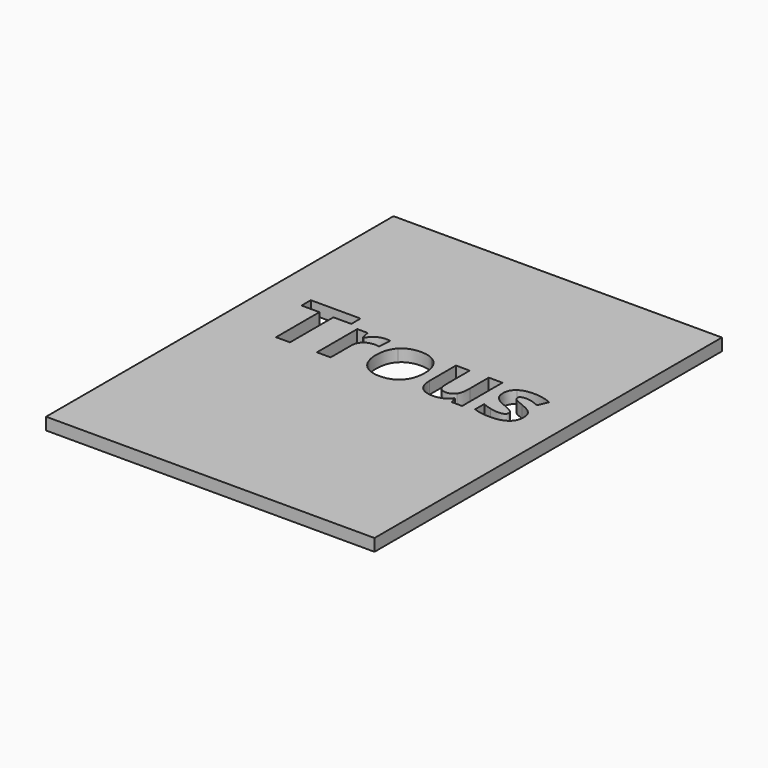
from build123d import *

# Parameters (mm, degrees)
F1_DEPTH = 10


# Not quite as in the source:
# - a feature names something its author has since deleted; it is built from what else it names


with BuildPart() as f1:
    # F0 (on Top) → F1 (new body)
    with BuildSketch(Plane.XY):
        Polygon((-135, 145.3171813515), (-135, -111.8657903795), (-105, -111.8657903795), (-105, 115.3171813515), (0, 115.3171813515), (0, 145.3171813515), align=None)
        Polygon((81.1492523154, -181.6828186485), (81.1492523154, -211.6828186485), (135, -211.6828186485), (135, -33.1828186485), (105, -33.1828186485), (105, -181.6828186485), align=None)
        Polygon((105, -33.1828186485), (135, -33.1828186485), (135, 145.3171813515), (0, 145.3171813515), (0, 115.3171813515), (105, 115.3171813515), (105, -20.8807700001), align=None)
        Polygon((-135, -111.8657903795), (-135, -211.6828186485), (81.1492523154, -211.6828186485), (81.1492523154, -181.6828186485), (-105, -181.6828186485), (-105, -111.8657903795), align=None)
        Polygon((-105, -181.6828186485), (81.1492523154, -181.6828186485), (105, -181.6828186485), (105, -33.1828186485), (105, -20.8807700001), (105, 115.3171813515), (0, 115.3171813515), (-105, 115.3171813515), (-105, -111.8657903795), align=None)
        Polygon((-77.2907613296, 11.4150706229), (-77.2907613296, -33.1828186485), (-88.7750437384, -33.1828186485), (-88.7750437384, 11.4150706229), (-103.4829843671, 11.4150706229), (-103.4829843671, 20.9675284366), (-62.5946723856, 20.9675284366), (-62.5946723856, 11.4150706229), align=None, mode=Mode.SUBTRACT)
        with BuildLine():
            add(Edge.make_bspline(
                [(-39.1698177098, 6.8699495664), (-35.892826909, 8.9973269579), (-32.0410294035, 8.9973269579)],
                knots=[0, 0, 0, 1, 1, 1], degree=2))
            add(Edge.make_bspline(
                [(-32.0410294035, 8.9973269579), (-29.7418025848, 8.9973269579), (-28.2247869519, 8.6654797882)],
                knots=[0, 0, 0, 1, 1, 1], degree=2))
            Line((-28.2247869519, 8.6654797882), (-29.0781082454, -1.9180745884))
            add(Edge.make_bspline(
                [(-29.0781082454, -1.9180745884), (-30.4529036627, -1.5506723648), (-32.4084316271, -1.5506723648)],
                knots=[0, 0, 0, 1, 1, 1], degree=2))
            add(Edge.make_bspline(
                [(-32.4084316271, -1.5506723648), (-37.8127998194, -1.5506723648), (-40.8349794006, -4.3298924111)],
                knots=[0, 0, 0, 1, 1, 1], degree=2))
            add(Edge.make_bspline(
                [(-40.8349794006, -4.3298924111), (-43.8571589819, -7.1091124574), (-43.8571589819, -12.1105233722)],
                knots=[0, 0, 0, 1, 1, 1], degree=2))
            Line((-43.8571589819, -12.1105233722), (-43.8571589819, -33.1828186485))
            Line((-43.8571589819, -33.1828186485), (-55.1518144365, -33.1828186485))
            Line((-55.1518144365, -33.1828186485), (-55.1518144365, 8.2269674568))
            Line((-55.1518144365, 8.2269674568), (-46.5948981319, 8.2269674568))
            Line((-46.5948981319, 8.2269674568), (-44.9238105988, 1.258176893))
            Line((-44.9238105988, 1.258176893), (-44.3786331057, 1.258176893))
            add(Edge.make_bspline(
                [(-44.3786331057, 1.258176893), (-42.4468085106, 4.7425721749), (-39.1698177098, 6.8699495664)],
                knots=[0, 0, 0, 1, 1, 1], degree=2))
        make_face(mode=Mode.SUBTRACT)
        with BuildLine():
            add(Edge.make_bspline(
                [(14.4768327784, -1.0351240833), (16.9182798126, -5.8883889403), (16.9182798126, -12.406815488)],
                knots=[0, 0, 0, 1, 1, 1], degree=2))
            add(Edge.make_bspline(
                [(16.9182798126, -12.406815488), (16.9182798126, -22.5163024794), (11.5850217281, -28.2228886299)],
                knots=[0, 0, 0, 1, 1, 1], degree=2))
            add(Edge.make_bspline(
                [(11.5850217281, -28.2228886299), (6.2517636435, -33.9294747803), (-3.2651391162, -33.9294747803)],
                knots=[0, 0, 0, 1, 1, 1], degree=2))
            add(Edge.make_bspline(
                [(-3.2651391162, -33.9294747803), (-9.2265364863, -33.9294747803), (-13.7835092274, -31.3161783189)],
                knots=[0, 0, 0, 1, 1, 1], degree=2))
            add(Edge.make_bspline(
                [(-13.7835092274, -31.3161783189), (-18.3404819685, -28.7028818575), (-20.7819290028, -23.8140619466)],
                knots=[0, 0, 0, 1, 1, 1], degree=2))
            add(Edge.make_bspline(
                [(-20.7819290028, -23.8140619466), (-23.223376037, -18.9252420358), (-23.223376037, -12.406815488)],
                knots=[0, 0, 0, 1, 1, 1], degree=2))
            add(Edge.make_bspline(
                [(-23.223376037, -12.406815488), (-23.223376037, -2.2617734428), (-17.9315988487, 3.3677767576)],
                knots=[0, 0, 0, 1, 1, 1], degree=2))
            add(Edge.make_bspline(
                [(-17.9315988487, 3.3677767576), (-12.6398216604, 8.9973269579), (-3.0399571082, 8.9973269579)],
                knots=[0, 0, 0, 1, 1, 1], degree=2))
            add(Edge.make_bspline(
                [(-3.0399571082, 8.9973269579), (2.9214402619, 8.9973269579), (7.478413003, 6.4077338658)],
                knots=[0, 0, 0, 1, 1, 1], degree=2))
            add(Edge.make_bspline(
                [(7.478413003, 6.4077338658), (12.0353857441, 3.8181407736), (14.4768327784, -1.0351240833)],
                knots=[0, 0, 0, 1, 1, 1], degree=2))
        make_face(mode=Mode.SUBTRACT)
        with BuildLine():
            Line((64.2539082341, -33.1828186485), (55.5903267679, -33.1828186485))
            Line((55.5903267679, -33.1828186485), (54.0733111349, -27.8851156178))
            Line((54.0733111349, -27.8851156178), (53.4807269033, -27.8851156178))
            add(Edge.make_bspline(
                [(53.4807269033, -27.8851156178), (51.6674191546, -30.7769266681), (48.3311699306, -32.3532007242)],
                knots=[0, 0, 0, 1, 1, 1], degree=2))
            add(Edge.make_bspline(
                [(48.3311699306, -32.3532007242), (44.9949207066, -33.9294747803), (40.7401659236, -33.9294747803)],
                knots=[0, 0, 0, 1, 1, 1], degree=2))
            add(Edge.make_bspline(
                [(40.7401659236, -33.9294747803), (33.4395281901, -33.9294747803), (29.7358767425, -30.0184188517)],
                knots=[0, 0, 0, 1, 1, 1], degree=2))
            add(Edge.make_bspline(
                [(29.7358767425, -30.0184188517), (26.0322252949, -26.107362923), (26.0322252949, -18.7711701356)],
                knots=[0, 0, 0, 1, 1, 1], degree=2))
            Line((26.0322252949, -18.7711701356), (26.0322252949, 8.2269674568))
            Line((26.0322252949, 8.2269674568), (37.3268807495, 8.2269674568))
            Line((37.3268807495, 8.2269674568), (37.3268807495, -15.9623208777))
            add(Edge.make_bspline(
                [(37.3268807495, -15.9623208777), (37.3268807495, -20.4422576688), (38.9209323325, -22.6822260643)],
                knots=[0, 0, 0, 1, 1, 1], degree=2))
            add(Edge.make_bspline(
                [(38.9209323325, -22.6822260643), (40.5149839156, -24.9221944598), (43.9993791975, -24.9221944598)],
                knots=[0, 0, 0, 1, 1, 1], degree=2))
            add(Edge.make_bspline(
                [(43.9993791975, -24.9221944598), (48.7400530504, -24.9221944598), (50.8496529149, -21.7577946629)],
                knots=[0, 0, 0, 1, 1, 1], degree=2))
            add(Edge.make_bspline(
                [(50.8496529149, -21.7577946629), (52.9592527795, -18.5933948661), (52.9592527795, -11.2572020787)],
                knots=[0, 0, 0, 1, 1, 1], degree=2))
            Line((52.9592527795, -11.2572020787), (52.9592527795, 8.2269674568))
            Line((52.9592527795, 8.2269674568), (64.2539082341, 8.2269674568))
            Line((64.2539082341, 8.2269674568), (64.2539082341, -33.1828186485))
        make_face(mode=Mode.SUBTRACT)
        with BuildLine():
            add(Edge.make_bspline(
                [(103.9214966985, -15.5889928118), (105, -17.8111836804), (105, -20.8807700001)],
                knots=[0, 0, 0, 1, 1, 1], degree=2))
            add(Edge.make_bspline(
                [(105, -20.8807700001), (105, -27.2569763323), (100.5733957898, -30.5932255563)],
                knots=[0, 0, 0, 1, 1, 1], degree=2))
            add(Edge.make_bspline(
                [(100.5733957898, -30.5932255563), (96.1467915797, -33.9294747803), (87.3291382132, -33.9294747803)],
                knots=[0, 0, 0, 1, 1, 1], degree=2))
            add(Edge.make_bspline(
                [(87.3291382132, -33.9294747803), (82.8136463683, -33.9294747803), (79.6255432022, -33.3131871794)],
                knots=[0, 0, 0, 1, 1, 1], degree=2))
            add(Edge.make_bspline(
                [(79.6255432022, -33.3131871794), (76.4374400361, -32.6968995786), (73.6641458322, -31.5117311153)],
                knots=[0, 0, 0, 1, 1, 1], degree=2))
            Line((73.6641458322, -31.5117311153), (73.6641458322, -22.1844553097))
            add(Edge.make_bspline(
                [(73.6641458322, -22.1844553097), (76.8048422597, -23.6659158887), (80.7514532423, -24.6673832402)],
                knots=[0, 0, 0, 1, 1, 1], degree=2))
            add(Edge.make_bspline(
                [(80.7514532423, -24.6673832402), (84.6980642248, -25.6688505916), (87.6965404368, -25.6688505916)],
                knots=[0, 0, 0, 1, 1, 1], degree=2))
            add(Edge.make_bspline(
                [(87.6965404368, -25.6688505916), (93.847564761, -25.6688505916), (93.847564761, -22.1133452019)],
                knots=[0, 0, 0, 1, 1, 1], degree=2))
            add(Edge.make_bspline(
                [(93.847564761, -22.1133452019), (93.847564761, -20.7741048385), (93.0297985214, -19.9385610719)],
                knots=[0, 0, 0, 1, 1, 1], degree=2))
            add(Edge.make_bspline(
                [(93.0297985214, -19.9385610719), (92.2120322817, -19.1030173053), (90.2150234212, -18.048217373)],
                knots=[0, 0, 0, 1, 1, 1], degree=2))
            add(Edge.make_bspline(
                [(90.2150234212, -18.048217373), (88.2180145606, -16.9934174408), (84.887691179, -15.5949186541)],
                knots=[0, 0, 0, 1, 1, 1], degree=2))
            add(Edge.make_bspline(
                [(84.887691179, -15.5949186541), (80.1114622721, -13.5919839513), (77.8655680343, -11.8853413642)],
                knots=[0, 0, 0, 1, 1, 1], degree=2))
            add(Edge.make_bspline(
                [(77.8655680343, -11.8853413642), (75.6196737965, -10.1786987772), (74.6063547604, -7.9742854356)],
                knots=[0, 0, 0, 1, 1, 1], degree=2))
            add(Edge.make_bspline(
                [(74.6063547604, -7.9742854356), (73.5930357244, -5.7698720939), (73.5930357244, -2.5580655586)],
                knots=[0, 0, 0, 1, 1, 1], degree=2))
            add(Edge.make_bspline(
                [(73.5930357244, -2.5580655586), (73.5930357244, 2.9648194801), (77.8655680343, 5.981073219)],
                knots=[0, 0, 0, 1, 1, 1], degree=2))
            add(Edge.make_bspline(
                [(77.8655680343, 5.981073219), (82.1381003443, 8.9973269579), (89.9957672555, 8.9973269579)],
                knots=[0, 0, 0, 1, 1, 1], degree=2))
            add(Edge.make_bspline(
                [(89.9957672555, 8.9973269579), (97.4741802585, 8.9973269579), (104.549635984, 5.738113684)],
                knots=[0, 0, 0, 1, 1, 1], degree=2))
            Line((104.549635984, 5.738113684), (101.1482024945, -2.4039936584))
            add(Edge.make_bspline(
                [(101.1482024945, -2.4039936584), (98.0312094362, -1.0766049796), (95.32902534, -0.223283686)],
                knots=[0, 0, 0, 1, 1, 1], degree=2))
            add(Edge.make_bspline(
                [(95.32902534, -0.223283686), (92.6268412439, 0.6300376075), (89.8061403014, 0.6300376075)],
                knots=[0, 0, 0, 1, 1, 1], degree=2))
            add(Edge.make_bspline(
                [(89.8061403014, 0.6300376075), (84.8047293865, 0.6300376075), (84.8047293865, -2.0721464887)],
                knots=[0, 0, 0, 1, 1, 1], degree=2))
            add(Edge.make_bspline(
                [(84.8047293865, -2.0721464887), (84.8047293865, -3.5891621216), (86.4165584965, -4.703220477)],
                knots=[0, 0, 0, 1, 1, 1], degree=2))
            add(Edge.make_bspline(
                [(86.4165584965, -4.703220477), (88.0283876065, -5.8172788325), (93.4801625374, -7.9979888048)],
                knots=[0, 0, 0, 1, 1, 1], degree=2))
            add(Edge.make_bspline(
                [(93.4801625374, -7.9979888048), (98.327501552, -9.9653684538), (100.5852474745, -11.6660851985)],
                knots=[0, 0, 0, 1, 1, 1], degree=2))
            add(Edge.make_bspline(
                [(100.5852474745, -11.6660851985), (102.8429933969, -13.3668019433), (103.9214966985, -15.5889928118)],
                knots=[0, 0, 0, 1, 1, 1], degree=2))
        make_face(mode=Mode.SUBTRACT)
    extrude(amount=F1_DEPTH)


solid = f1.part
